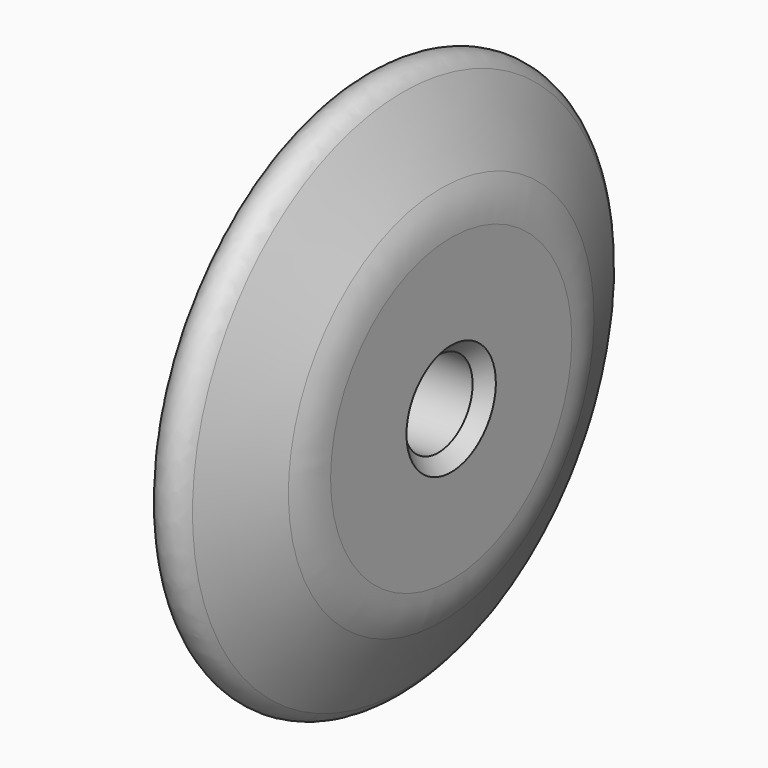
from build123d import *

# Parameters (mm, degrees)
F0_W    = 30
F0_H    = 30
F7_R    = 5
F1_R    = 20
F2_SIZE = 3


# Not quite as in the source:
# - the program builds the solid bodies; features that only make, move or delete a surface that nothing else refers to are left out


with BuildPart() as f6:
    # F0 (on Front) → F6 (revolve)
    with BuildSketch(Plane.XZ):
        Polygon((-34.5531404018, 69.9733775854), (-48.6977283961, 39.9733775854), (-18.6977283961, 39.9733775854), align=None)
        with Locations((-33.6977283961, 24.9733775854)):
            Rectangle(F0_W, F0_H)
    revolve(axis=Axis((8.8008791208, 0, 0), (1, 0, 0)))

    # F7
    f7_edges = [f6.edges().sort_by_distance(p)[0] for p in [
        (-34.55314, 0, -69.973378),
    ]]
    fillet(f7_edges, radius=F7_R)

    # F1
    f1_edges = [f6.edges().sort_by_distance(p)[0] for p in [
        (-18.697728, 0, -39.973378),
    ]]
    fillet(f1_edges, radius=F1_R)

    # F2
    f2_edges = [f6.edges().sort_by_distance(p)[0] for p in [
        (-18.697728, 0, -9.973378),
    ]]
    chamfer(f2_edges, length=F2_SIZE)


solid = f6.part
